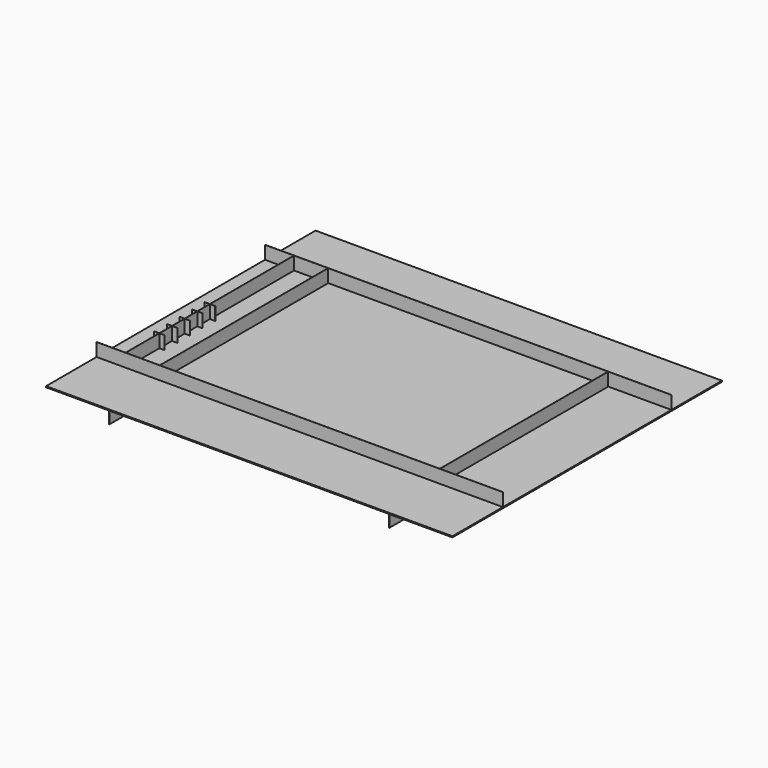
from build123d import *

# Parameters (mm, degrees)
F0_W     = 772
F0_H     = 640
F1_DEPTH = 2
F2_W     = 0.25
F2_H     = 119.9
F3_DEPTH = 25
F4_DEPTH = 25
F2_W_2   = 119.9
F2_H_2   = 0.2
F2_W_3   = 0.2
F2_H_3   = 399.8
F5_DEPTH = 25
F2_W_4   = 64.7
F6_DEPTH = 25
F2_W_5   = 55
F7_DEPTH = 25
F2_H_4   = 49.5626640439
F8_DEPTH = 25
F2_H_5   = 199.6
F2_W_6   = 9.8
F2_H_6   = 30.4373359561
F2_W_7   = 10
F2_H_7   = 29.8
F9_DEPTH = 25


# Not quite as in the source:
# - a feature names something its author has since deleted; it is built from what else it names


with BuildPart() as f1:
    # F0 (on Top) → F1 (new body)
    with BuildSketch(Plane.XY):
        with Locations((386, 320)):
            Rectangle(F0_W, F0_H)
    extrude(amount=F1_DEPTH)

    # F2 (on face) → F3 (join)
    with BuildSketch(Plane.XY.offset(2)):
        with Locations((651.975, 580.05)):
            Rectangle(F2_W, F2_H)
        with Locations((120.025, 580.05)):
            Rectangle(F2_W, F2_H)
        Polygon((120.1, 119.9), (119.9, 119.9), (119.9, 0), (120.15, 0), (120.15, 119.9), align=None)
        Polygon((652.1, 119.9), (651.9, 119.9), (651.85, 119.9), (651.85, 0), (652.1, 0), align=None)
    extrude(amount=-F3_DEPTH)

    # F2 (on face) → F4 (join)
    with BuildSketch(Plane.XY.offset(2)):
        Polygon((119.9, 520.1), (0, 520.1), (0, 519.9), (55, 519.9), (55.2, 519.9), (119.9, 519.9), align=None)
        Polygon((651.85, 520.1), (120.15, 520.1), (120.15, 519.9), (651.9, 519.9), (652.1, 519.9), (652.1, 520.1), align=None)
    extrude(amount=F4_DEPTH)

    # F2 (on face) → F5 (join)
    with BuildSketch(Plane.XY.offset(2)):
        with Locations((712.05, 520)):
            Rectangle(F2_W_2, F2_H_2)
        with Locations((652, 320)):
            Rectangle(F2_W_3, F2_H_3)
    extrude(amount=F5_DEPTH)

    # F2 (on face) → F6 (join)
    with BuildSketch(Plane.XY.offset(2)):
        with Locations((712.05, 120)):
            Rectangle(F2_W_2, F2_H_2)
        Polygon((651.9, 120.1), (120.1, 120.1), (120.1, 119.9), (120.15, 119.9), (651.85, 119.9), (651.9, 119.9), align=None)
        with Locations((652, 120)):
            Rectangle(F2_W_3, F2_H_2)
        with Locations((87.55, 120)):
            Rectangle(F2_W_4, F2_H_2)
        with Locations((120, 120)):
            Rectangle(F2_W_3, F2_H_2)
    extrude(amount=F6_DEPTH)

    # F2 (on face) → F7 (join)
    with BuildSketch(Plane.XY.offset(2)):
        with Locations((27.5, 120)):
            Rectangle(F2_W_5, F2_H_2)
    extrude(amount=F7_DEPTH)

    # F2 (on face) → F8 (join)
    with BuildSketch(Plane.XY.offset(2)):
        with Locations((55.1, 175.318667978)):
            Rectangle(F2_W_3, F2_H_4)
    extrude(amount=F8_DEPTH)

    # F2 (on face) → F9 (join)
    with BuildSketch(Plane.XY.offset(2)):
        Polygon((120.15, 520.1), (119.9, 520.1), (119.9, 519.9), (120.1, 519.9), (120.15, 519.9), align=None)
        with Locations((120, 320)):
            Rectangle(F2_W_3, F2_H_3)
        with Locations((55.1, 420.1)):
            Rectangle(F2_W_3, F2_H_5)
        with Locations((55.1, 320.2)):
            Rectangle(F2_W_3, F2_H_2)
        with Locations((50.1, 320.2)):
            Rectangle(F2_W_6, F2_H_2)
        with Locations((55.1, 135.318667978)):
            Rectangle(F2_W_3, F2_H_6)
        with Locations((55.1, 120)):
            Rectangle(F2_W_3, F2_H_2)
        with Locations((60.2, 320.2)):
            Rectangle(F2_W_7, F2_H_2)
        with Locations((55.1, 305.2)):
            Rectangle(F2_W_3, F2_H_7)
        with Locations((55.1, 175.318667978)):
            Rectangle(F2_W_3, F2_H_4)
        with Locations((55.1, 290.2)):
            Rectangle(F2_W_3, F2_H_2)
        with Locations((50.1, 290.2)):
            Rectangle(F2_W_6, F2_H_2)
        with Locations((50.1, 200.2)):
            Rectangle(F2_W_6, F2_H_2)
        with Locations((55.1, 200.2)):
            Rectangle(F2_W_3, F2_H_2)
        with Locations((60.2, 290.2)):
            Rectangle(F2_W_7, F2_H_2)
        with Locations((60.2, 200.2)):
            Rectangle(F2_W_7, F2_H_2)
        with Locations((55.1, 275.2)):
            Rectangle(F2_W_3, F2_H_7)
        with Locations((55.1, 215.2)):
            Rectangle(F2_W_3, F2_H_7)
        with Locations((55.1, 260.2)):
            Rectangle(F2_W_3, F2_H_2)
        with Locations((50.1, 260.2)):
            Rectangle(F2_W_6, F2_H_2)
        with Locations((50.1, 230.2)):
            Rectangle(F2_W_6, F2_H_2)
        with Locations((55.1, 230.2)):
            Rectangle(F2_W_3, F2_H_2)
        with Locations((60.2, 260.2)):
            Rectangle(F2_W_7, F2_H_2)
        with Locations((60.2, 230.2)):
            Rectangle(F2_W_7, F2_H_2)
        with Locations((55.1, 245.2)):
            Rectangle(F2_W_3, F2_H_7)
    extrude(amount=F9_DEPTH)


solid = f1.part
